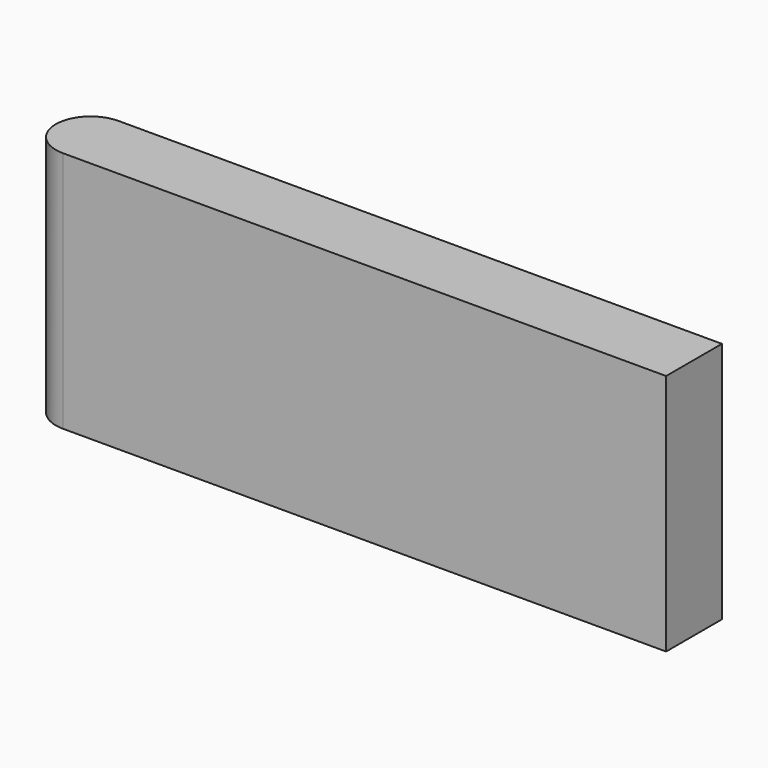
from build123d import *

# Parameters (mm, degrees)
F0_W     = 116.2035912275
F0_H     = 44.1677831113
F1_DEPTH = 12.7
F2_R     = 6.34999


# Not quite as in the source:
# - a fillet or chamfer is up to 0.001 mm smaller than in the source, because OpenCascade refuses the exact size


with BuildPart() as f1:
    # F0 (on Front) → F1 (new body)
    with BuildSketch(Plane.XZ):
        Rectangle(F0_W, F0_H)
    extrude(amount=F1_DEPTH)

    # F2 (radius 6.35 in the source; OpenCascade refuses exactly that, so slightly less here)
    f2_edges = [f1.edges().sort_by_distance(p)[0] for p in [
        (-58.101796, 0, 0),
        (-58.101796, -12.7, 0),
    ]]
    fillet(f2_edges, radius=F2_R)


solid = f1.part
